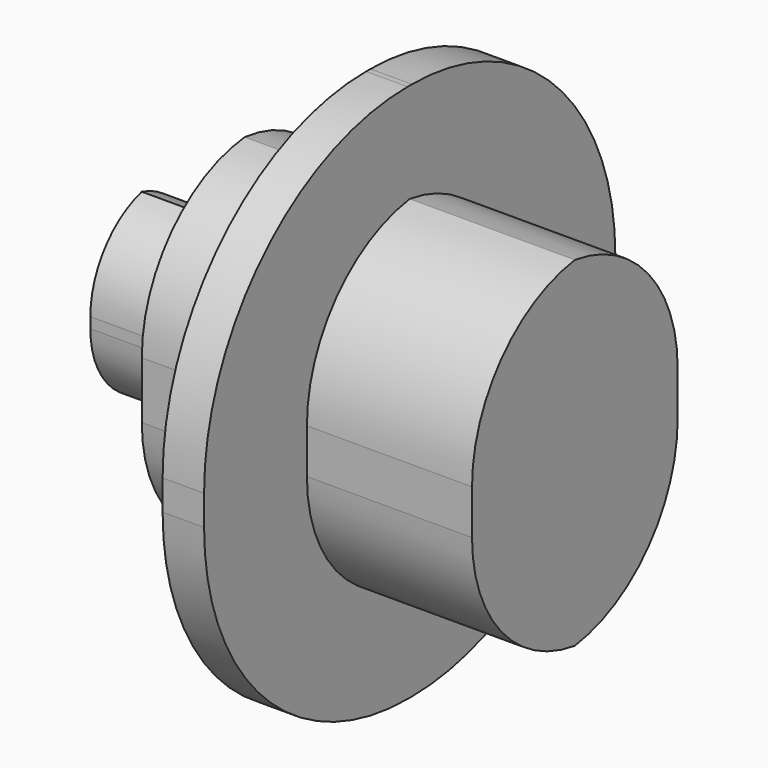
from build123d import *

# Parameters (mm, degrees)
F1_DEPTH    = 25.4
F2_DEPTH    = 12.7
F3_DEPTH    = 6.35
F4_T1_DEPTH = 31.6265151256
F5_T1_DEPTH = 12.2162196785
F6_R        = 25.1416200386
F7_T1_DEPTH = 53.1085051667


# Not quite as in the source:
# - a fillet or chamfer that OpenCascade refuses, or shapes differently, is made with other operations: its cross-section is extruded or revolved along the edge and cut away or added


with BuildPart() as f1:
    # F0 (on Front) → F1 (new body, symmetric)
    with BuildSketch(Plane.XZ):
        Polygon((-20.4155612737, 26.5935901552), (-20.4155612737, 16.8710052967), (-20.4155612737, -16.9768668711), (-20.4155612737, -26.6668144614), (-16.3158904761, -26.6668144614), (-16.3158904761, -16.9768668711), (-16.3158904761, 16.8710052967), (-16.3158904761, 26.5935901552), align=None)
    extrude(amount=F1_DEPTH, both=True)

    # F0 (on Front) → F2 (join, symmetric)
    with BuildSketch(Plane.XZ):
        Polygon((-32.6317809522, 16.8710052967), (-32.6317809522, 9.0427109972), (-32.6317809522, -9.1775488108), (-32.6317809522, -16.9768668711), (-20.4155612737, -16.9768668711), (-20.4155612737, 16.8710052967), align=None)
        Polygon((0, 16.8710052967), (-16.3158904761, 16.8710052967), (-16.3158904761, -16.9768668711), (0, -16.9768668711), (0, -9.1775488108), (0, 0), (0, 9.0427109972), align=None)
    extrude(amount=F2_DEPTH, both=True)

    # F0 (on Front) → F3 (join, symmetric)
    with BuildSketch(Plane.XZ):
        Polygon((-32.6317809522, -9.1775488108), (-32.6317809522, 9.0427109972), (-42.7959375083, 9.0427109972), (-42.7959375083, 0), (-42.7959375083, -9.1775488108), align=None)
    extrude(amount=F3_DEPTH, both=True)

    # F4: fillet of radius 8.5849434278 on 4 edges, made by hand

    # F4_s2 → F4_t1 (cut)
    with BuildSketch(Plane.YZ.offset(-64.2582960778)):
        with BuildLine():
            ThreePointArc((-6.35, 0.4577675694), (-3.8355282861, 6.5282392833), (2.2349434278, 9.0427109972))
            Line((2.2349434278, 9.0427109972), (-6.35, 9.0427109972))
            Line((-6.35, 9.0427109972), (-6.35, 0.4577675694))
        make_face()
        with BuildLine():
            ThreePointArc((2.2349434278, -9.1775488108), (-3.8355282861, -6.6630770969), (-6.35, -0.592605383))
            Line((-6.35, -0.592605383), (-6.35, -9.1775488108))
            Line((-6.35, -9.1775488108), (2.2349434278, -9.1775488108))
        make_face()
        with BuildLine():
            ThreePointArc((-2.2349434278, 9.0427109972), (3.8355282861, 6.5282392833), (6.35, 0.4577675694))
            Line((6.35, 0.4577675694), (6.35, 9.0427109972))
            Line((6.35, 9.0427109972), (-2.2349434278, 9.0427109972))
        make_face()
        with BuildLine():
            ThreePointArc((-2.2349434278, -9.1775488108), (3.8355282861, -6.6630770969), (6.35, -0.592605383))
            Line((6.35, -0.592605383), (6.35, -9.1775488108))
            Line((6.35, -9.1775488108), (-2.2349434278, -9.1775488108))
        make_face()
    extrude(amount=F4_T1_DEPTH, mode=Mode.SUBTRACT)

    # F5: fillet of radius 14.1038356314 on 4 edges, made by hand

    # F5_s2 → F5_t1 (cut)
    with BuildSketch(Plane.YZ.offset(-32.6317809522)):
        with BuildLine():
            ThreePointArc((-1.4038356314, 16.8710052967), (8.5690821843, 12.740087481), (12.7, 2.7671696653))
            Line((12.7, 2.7671696653), (12.9820767126, 2.7671696653))
            Line((12.9820767126, 2.7671696653), (12.9820767126, 17.1530820093))
            Line((12.9820767126, 17.1530820093), (-1.4038356314, 17.1530820093))
            Line((-1.4038356314, 17.1530820093), (-1.4038356314, 16.8710052967))
        make_face()
        with BuildLine():
            ThreePointArc((12.7, -2.8730312397), (8.5690821843, -12.8459490554), (-1.4038356314, -16.9768668711))
            Line((-1.4038356314, -16.9768668711), (-1.4038356314, -17.2589435837))
            Line((-1.4038356314, -17.2589435837), (12.9820767126, -17.2589435837))
            Line((12.9820767126, -17.2589435837), (12.9820767126, -2.8730312397))
            Line((12.9820767126, -2.8730312397), (12.7, -2.8730312397))
        make_face()
        with BuildLine():
            ThreePointArc((1.4038356314, 16.8710052967), (-8.5690821843, 12.740087481), (-12.7, 2.7671696653))
            Line((-12.7, 2.7671696653), (-12.9820767126, 2.7671696653))
            Line((-12.9820767126, 2.7671696653), (-12.9820767126, 17.1530820093))
            Line((-12.9820767126, 17.1530820093), (1.4038356314, 17.1530820093))
            Line((1.4038356314, 17.1530820093), (1.4038356314, 16.8710052967))
        make_face()
        with BuildLine():
            ThreePointArc((1.4038356314, -16.9768668711), (-8.5690821843, -12.8459490554), (-12.7, -2.8730312397))
            Line((-12.7, -2.8730312397), (-12.9820767126, -2.8730312397))
            Line((-12.9820767126, -2.8730312397), (-12.9820767126, -17.2589435837))
            Line((-12.9820767126, -17.2589435837), (1.4038356314, -17.2589435837))
            Line((1.4038356314, -17.2589435837), (1.4038356314, -16.9768668711))
        make_face()
    extrude(amount=F5_T1_DEPTH, mode=Mode.SUBTRACT)

    # F6
    f6_edges = [f1.edges().sort_by_distance(p)[0] for p in [
        (-18.365726, -25.4, 26.59359),
        (-18.365726, -25.4, -26.666814),
        (-18.365726, 25.4, 26.59359),
        (-18.365726, 25.4, -26.666814),
    ]]
    fillet(f6_edges, radius=F6_R)

    # F7: fillet of radius 14.7170458762 on 4 edges, made by hand

    # F7_s2 → F7_t1 (cut)
    with BuildSketch(Plane.YZ.offset(-16.3158904761)):
        with BuildLine():
            ThreePointArc((-2.0170458762, 16.8710052967), (8.3894770619, 12.5604823586), (12.7, 2.1539594205))
            Line((12.7, 2.1539594205), (12.7, 16.8710052967))
            Line((12.7, 16.8710052967), (-2.0170458762, 16.8710052967))
        make_face()
        with BuildLine():
            ThreePointArc((-2.0170458762, -16.9768668711), (8.3894770619, -12.666343933), (12.7, -2.2598209949))
            Line((12.7, -2.2598209949), (12.7, -16.9768668711))
            Line((12.7, -16.9768668711), (-2.0170458762, -16.9768668711))
        make_face()
        with BuildLine():
            ThreePointArc((2.0170458762, 16.8710052967), (-8.3894770619, 12.5604823586), (-12.7, 2.1539594205))
            Line((-12.7, 2.1539594205), (-12.7, 16.8710052967))
            Line((-12.7, 16.8710052967), (2.0170458762, 16.8710052967))
        make_face()
        with BuildLine():
            ThreePointArc((-12.7, -2.2598209949), (-8.3894770619, -12.666343933), (2.0170458762, -16.9768668711))
            Line((2.0170458762, -16.9768668711), (-12.7, -16.9768668711))
            Line((-12.7, -16.9768668711), (-12.7, -2.2598209949))
        make_face()
    extrude(amount=F7_T1_DEPTH, mode=Mode.SUBTRACT)


solid = f1.part
